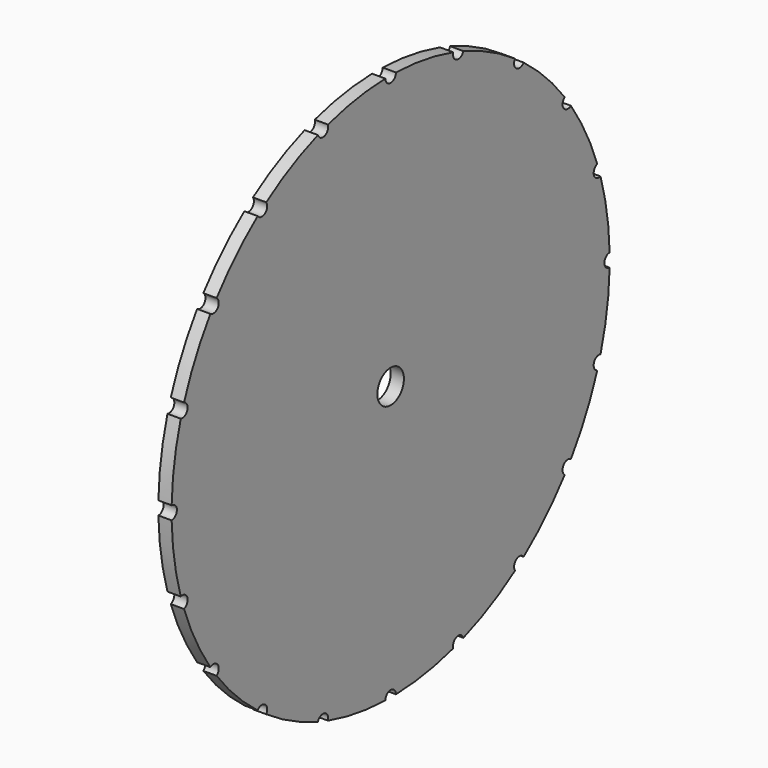
from build123d import *

# Parameters (mm, degrees)
F0_R            = 82.5
F0_R_2          = 5
F1_DEPTH        = 2
F1_DEPTH_BACK   = 2
F2_R            = 2
F3_DEPTH        = 4.001
F3_COPIES_COUNT = 20


# Not quite as in the source:
# - a pattern or mirror of a feature is missing from the dataset's text; its kind, count and spacing are read off the source's solid


with BuildPart() as f1:
    # F0 (on Right) → F1 (new body, two sides)
    with BuildSketch(Plane.YZ) as f1_sk:
        Circle(F0_R)
        Circle(F0_R_2, mode=Mode.SUBTRACT)
    extrude(amount=F1_DEPTH)
    extrude(f1_sk.sketch, amount=-F1_DEPTH_BACK)

    # F2 (on face) → F3 (cut, through all)
    with BuildSketch(Plane.YZ.offset(2)):
        with Locations((0, 82.5)):
            Circle(F2_R)
    f3 = extrude(amount=-F3_DEPTH, mode=Mode.SUBTRACT)

    # F3_copies: F3 ×20 about axis
    f3_copies_axis = Axis((0, 0, 0), (1, 0, 0))
    for i in range(1, F3_COPIES_COUNT):
        add(f3.rotate(f3_copies_axis, i * 360 / F3_COPIES_COUNT), mode=Mode.SUBTRACT)


solid = f1.part
